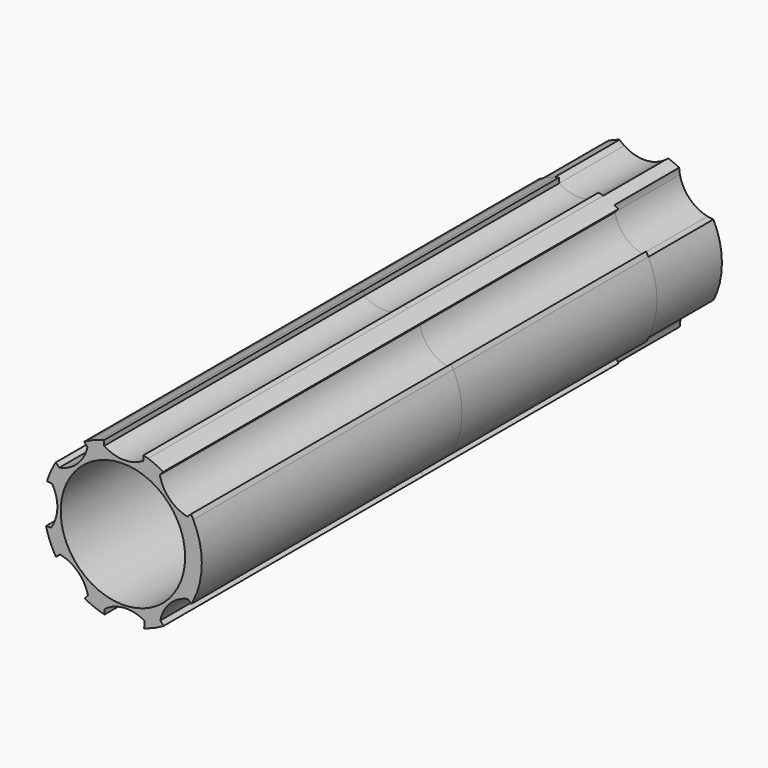
from build123d import *

# Parameters (mm, degrees)
F0_R          = 4.8612376023
F1_DEPTH      = 25.4
F1_DEPTH_BACK = 25.4
F2_DEPTH      = 19.05
F2_DEPTH_BACK = 25.4
F3_DEPTH      = 25.4
F3_DEPTH_BACK = 25.4
F4_T2_ANGLE   = 271.2368100282


# Not quite as in the source:
# - a fillet or chamfer that OpenCascade refuses, or shapes differently, is made with other operations: its cross-section is extruded or revolved along the edge and cut away or added


with BuildPart() as f1:
    # F0 (on Front) → F1 (new body, two sides)
    with BuildSketch(Plane.XZ) as f1_sk:
        with BuildLine():
            ThreePointArc((-5.6143828163, -1.3793864731), (-5.7555397167, -1.5672020545), (-5.9119525631, -1.7425160147))
            ThreePointArc((-5.9119525631, -1.7425160147), (-5.6940196105, -2.3591705842), (-5.4119693183, -2.9492597831))
            ThreePointArc((-5.4119693183, -2.9492597831), (-5.1782834381, -2.962493255), (-4.9465206336, -2.9952074382))
            ThreePointArc((-4.9465206336, -2.9952074382), (-3.5276076708, -3.7167374387), (-2.7316714584, -5.0952892453))
            ThreePointArc((-2.7316714584, -5.0952892453), (-2.6865496833, -5.3258624193), (-2.6609266437, -5.5594077533))
            ThreePointArc((-2.6609266437, -5.5594077533), (-2.2164022319, -5.751096097), (-1.7582047643, -5.907305746))
            ThreePointArc((-1.7582047643, -5.907305746), (-1.5960910736, -5.7494322847), (-1.4217527636, -5.6051719916))
            ThreePointArc((-1.4217527636, -5.6051719916), (0.114197137, -5.0376327164), (1.7047800347, -5.4265915467))
            Line((1.7047800347, -5.4265915467), (1.6597306544, -5.935725678))
            ThreePointArc((1.6597306544, -5.935725678), (2.2765492286, -5.7275534725), (2.8679699144, -5.4554829062))
            ThreePointArc((2.8679699144, -5.4554829062), (2.8846977078, -5.22202114), (2.9208752645, -4.990773654))
            ThreePointArc((2.9208752645, -4.990773654), (3.6635506236, -3.582813126), (5.0538549065, -2.807588295))
            ThreePointArc((5.0538549065, -2.807588295), (5.2850772748, -2.7659208069), (5.5189797809, -2.7437943341))
            ThreePointArc((5.5189797809, -2.7437943341), (6.1633583889, 0.023633466), (5.4977755768, 2.7860382045))
            ThreePointArc((5.4977755768, 2.7860382045), (5.2645901724, 2.8062565756), (5.0339097574, 2.8458894094))
            ThreePointArc((5.0339097574, 2.8458894094), (3.6372167606, 3.6095439191), (2.8828768034, 5.0112895332))
            ThreePointArc((2.8828768034, 5.0112895332), (2.8446729274, 5.2431093491), (2.8260479734, 5.4773166809))
            ThreePointArc((2.8260479734, 5.4773166809), (2.4006224975, 5.6766677545), (1.961248138, 5.8430343924))
            ThreePointArc((1.961248138, 5.8430343924), (1.7809432193, 5.6937884489), (1.588797766, 5.5601309009))
            ThreePointArc((1.588797766, 5.5601309009), (0.0578959269, 5.1239439038), (-1.4632199599, 5.5931197733))
            ThreePointArc((-1.4632199599, 5.5931197733), (-1.6531261487, 5.7314512688), (-1.830760335, 5.88522402))
            ThreePointArc((-1.830760335, 5.88522402), (-2.2737274404, 5.728674253), (-2.7034829894, 5.5388378651))
            ThreePointArc((-2.7034829894, 5.5388378651), (-2.7271874135, 5.3059810086), (-2.7702666546, 5.07591929))
            ThreePointArc((-2.7702666546, 5.07591929), (-3.5547294118, 3.6908063992), (-4.9676026515, 2.9575201346))
            ThreePointArc((-4.9676026515, 2.9575201346), (-5.1999680345, 2.9227884204), (-5.4344277772, 2.9076691533))
            ThreePointArc((-5.4344277772, 2.9076691533), (-5.6401206566, 2.4852734556), (-5.8130414583, 2.0484370076))
            ThreePointArc((-5.8130414583, 2.0484370076), (-5.6665094698, 1.8659196339), (-5.5357412598, 1.6717962436))
            ThreePointArc((-5.5357412598, 1.6717962436), (-5.122504455, 0.1345406108), (-5.6143828163, -1.3793864731))
        make_face()
        Circle(F0_R, mode=Mode.SUBTRACT)
    extrude(amount=-F1_DEPTH)
    extrude(f1_sk.sketch, amount=F1_DEPTH_BACK)

    # F0 (on Front) → F2 (join, two sides)
    with BuildSketch(Plane.XZ) as f2_sk:
        with BuildLine():
            ThreePointArc((3.1433341705, 5.3016031031), (2.9859838597, 5.3917942802), (2.8260479734, 5.4773166809))
            ThreePointArc((2.8260479734, 5.4773166809), (2.8446729274, 5.2431093491), (2.8828768034, 5.0112895332))
            Line((2.8828768034, 5.0112895332), (3.1433341705, 5.3016031031))
        make_face()
        with BuildLine():
            Line((1.6092045641, 5.9496223276), (1.588797766, 5.5601309009))
            ThreePointArc((1.588797766, 5.5601309009), (1.7809432193, 5.6937884489), (1.961248138, 5.8430343924))
            ThreePointArc((1.961248138, 5.8430343924), (1.7860216604, 5.8989551447), (1.6092045641, 5.9496223276))
        make_face()
        with BuildLine():
            ThreePointArc((-1.4814178118, 5.9827206551), (-1.6568063911, 5.9365425757), (-1.830760335, 5.88522402))
            ThreePointArc((-1.830760335, 5.88522402), (-1.6531261487, 5.7314512688), (-1.4632199599, 5.5931197733))
            Line((-1.4632199599, 5.5931197733), (-1.4814178118, 5.9827206551))
        make_face()
        with BuildLine():
            Line((-3.0290736059, 5.3677051205), (-2.7702666546, 5.07591929))
            ThreePointArc((-2.7702666546, 5.07591929), (-2.7271874135, 5.3059810086), (-2.7034829894, 5.5388378651))
            ThreePointArc((-2.7034829894, 5.5388378651), (-2.8675552102, 5.4557008978), (-3.0290736059, 5.3677051205))
        make_face()
        with BuildLine():
            ThreePointArc((-5.253987448, 3.2222912758), (-5.3465224003, 3.0663077787), (-5.4344277772, 2.9076691533))
            ThreePointArc((-5.4344277772, 2.9076691533), (-5.1999680345, 2.9227884204), (-4.9676026515, 2.9575201346))
            Line((-4.9676026515, 2.9575201346), (-5.253987448, 3.2222912758))
        make_face()
        with BuildLine():
            Line((-5.9248838296, 1.698027319), (-5.5357412598, 1.6717962436))
            ThreePointArc((-5.5357412598, 1.6717962436), (-5.6665094698, 1.8659196339), (-5.8130414583, 2.0484370076))
            ThreePointArc((-5.8130414583, 2.0484370076), (-5.8715772373, 1.8740666788), (-5.9248838296, 1.698027319))
        make_face()
        with BuildLine():
            ThreePointArc((-6.0042123315, -1.3917540905), (-5.9606631284, -1.5678138408), (-5.9119525631, -1.7425160147))
            ThreePointArc((-5.9119525631, -1.7425160147), (-5.7555397167, -1.5672020545), (-5.6143828163, -1.3793864731))
            Line((-5.6143828163, -1.3793864731), (-6.0042123315, -1.3917540905))
        make_face()
        with BuildLine():
            ThreePointArc((5.0339097574, 2.8458894094), (5.2645901724, 2.8062565756), (5.4977755768, 2.7860382045))
            ThreePointArc((5.4977755768, 2.7860382045), (5.4121934892, 2.9488483863), (5.321791339, 3.1090323437))
            Line((5.321791339, 3.1090323437), (5.0339097574, 2.8458894094))
        make_face()
        with BuildLine():
            ThreePointArc((5.5189797809, -2.7437943341), (5.2850772748, -2.7659208069), (5.0538549065, -2.807588295))
            Line((5.0538549065, -2.807588295), (5.3480322785, -3.0636735985))
            ThreePointArc((5.3480322785, -3.0636735985), (5.4358594961, -2.9049916883), (5.5189797809, -2.7437943341))
        make_face()
        with BuildLine():
            ThreePointArc((2.9208752645, -4.990773654), (2.8846977078, -5.22202114), (2.8679699144, -5.4554829062))
            ThreePointArc((2.8679699144, -5.4554829062), (3.0294816207, -5.3674748514), (3.1882952913, -5.27468656))
            Line((3.1882952913, -5.27468656), (2.9208752645, -4.990773654))
        make_face()
        with BuildLine():
            ThreePointArc((-5.6143828163, -1.3793864731), (-5.7555397167, -1.5672020545), (-5.9119525631, -1.7425160147))
            ThreePointArc((-5.9119525631, -1.7425160147), (-5.6940196105, -2.3591705842), (-5.4119693183, -2.9492597831))
            ThreePointArc((-5.4119693183, -2.9492597831), (-5.1782834381, -2.962493255), (-4.9465206336, -2.9952074382))
            ThreePointArc((-4.9465206336, -2.9952074382), (-3.5276076708, -3.7167374387), (-2.7316714584, -5.0952892453))
            ThreePointArc((-2.7316714584, -5.0952892453), (-2.6865496833, -5.3258624193), (-2.6609266437, -5.5594077533))
            ThreePointArc((-2.6609266437, -5.5594077533), (-2.2164022319, -5.751096097), (-1.7582047643, -5.907305746))
            ThreePointArc((-1.7582047643, -5.907305746), (-1.5960910736, -5.7494322847), (-1.4217527636, -5.6051719916))
            ThreePointArc((-1.4217527636, -5.6051719916), (0.114197137, -5.0376327164), (1.7047800347, -5.4265915467))
            Line((1.7047800347, -5.4265915467), (1.6597306544, -5.935725678))
            ThreePointArc((1.6597306544, -5.935725678), (2.2765492286, -5.7275534725), (2.8679699144, -5.4554829062))
            ThreePointArc((2.8679699144, -5.4554829062), (2.8846977078, -5.22202114), (2.9208752645, -4.990773654))
            ThreePointArc((2.9208752645, -4.990773654), (3.6635506236, -3.582813126), (5.0538549065, -2.807588295))
            ThreePointArc((5.0538549065, -2.807588295), (5.2850772748, -2.7659208069), (5.5189797809, -2.7437943341))
            ThreePointArc((5.5189797809, -2.7437943341), (6.1633583889, 0.023633466), (5.4977755768, 2.7860382045))
            ThreePointArc((5.4977755768, 2.7860382045), (5.2645901724, 2.8062565756), (5.0339097574, 2.8458894094))
            ThreePointArc((5.0339097574, 2.8458894094), (3.6372167606, 3.6095439191), (2.8828768034, 5.0112895332))
            ThreePointArc((2.8828768034, 5.0112895332), (2.8446729274, 5.2431093491), (2.8260479734, 5.4773166809))
            ThreePointArc((2.8260479734, 5.4773166809), (2.4006224975, 5.6766677545), (1.961248138, 5.8430343924))
            ThreePointArc((1.961248138, 5.8430343924), (1.7809432193, 5.6937884489), (1.588797766, 5.5601309009))
            ThreePointArc((1.588797766, 5.5601309009), (0.0578959269, 5.1239439038), (-1.4632199599, 5.5931197733))
            ThreePointArc((-1.4632199599, 5.5931197733), (-1.6531261487, 5.7314512688), (-1.830760335, 5.88522402))
            ThreePointArc((-1.830760335, 5.88522402), (-2.2737274404, 5.728674253), (-2.7034829894, 5.5388378651))
            ThreePointArc((-2.7034829894, 5.5388378651), (-2.7271874135, 5.3059810086), (-2.7702666546, 5.07591929))
            ThreePointArc((-2.7702666546, 5.07591929), (-3.5547294118, 3.6908063992), (-4.9676026515, 2.9575201346))
            ThreePointArc((-4.9676026515, 2.9575201346), (-5.1999680345, 2.9227884204), (-5.4344277772, 2.9076691533))
            ThreePointArc((-5.4344277772, 2.9076691533), (-5.6401206566, 2.4852734556), (-5.8130414583, 2.0484370076))
            ThreePointArc((-5.8130414583, 2.0484370076), (-5.6665094698, 1.8659196339), (-5.5357412598, 1.6717962436))
            ThreePointArc((-5.5357412598, 1.6717962436), (-5.122504455, 0.1345406108), (-5.6143828163, -1.3793864731))
        make_face()
        Circle(F0_R, mode=Mode.SUBTRACT)
        with BuildLine():
            ThreePointArc((-1.4217527636, -5.6051719916), (-1.5960910736, -5.7494322847), (-1.7582047643, -5.907305746))
            ThreePointArc((-1.7582047643, -5.907305746), (-1.5949558747, -5.9534578967), (-1.4304986106, -5.9950995734))
            Line((-1.4304986106, -5.9950995734), (-1.4217527636, -5.6051719916))
        make_face()
        with BuildLine():
            ThreePointArc((-2.6609266437, -5.5594077533), (-2.6865496833, -5.3258624193), (-2.7316714584, -5.0952892453))
            Line((-2.7316714584, -5.0952892453), (-2.9833273874, -5.3932645837))
            ThreePointArc((-2.9833273874, -5.3932645837), (-2.8233493903, -5.4787081863), (-2.6609266437, -5.5594077533))
        make_face()
        with BuildLine():
            ThreePointArc((-4.9465206336, -2.9952074382), (-5.1782834381, -2.962493255), (-5.4119693183, -2.9492597831))
            ThreePointArc((-5.4119693183, -2.9492597831), (-5.321554992, -3.1094368681), (-5.2264013251, -3.2668447099))
            Line((-5.2264013251, -3.2668447099), (-4.9465206336, -2.9952074382))
        make_face()
    extrude(amount=-F2_DEPTH)
    extrude(f2_sk.sketch, amount=F2_DEPTH_BACK)


with BuildPart() as f3:
    # F0 (on Front) → F3 (new body, two sides)
    with BuildSketch(Plane.XZ) as f3_sk:
        with BuildLine():
            Line((-1.3347425842, -5.6051719916), (-1.3347425842, -5.8972059093))
            ThreePointArc((-1.3347425842, -5.8972059093), (0.1551903565, -6.0448676148), (1.63668259, -5.8283383814))
            Line((1.63668259, -5.8283383814), (1.6722300908, -5.4265915467))
            ThreePointArc((1.6722300908, -5.4265915467), (0.1408736066, -5.0465987547), (-1.3347425842, -5.6051719916))
        make_face()
    extrude(amount=-F3_DEPTH)
    extrude(f3_sk.sketch, amount=F3_DEPTH_BACK)

    # F4: chamfer of 5.08 on 1 edges, made by hand

    # F4_s1 → F4_t2 (revolve, cut)
    with BuildSketch(Plane(origin=(0.0596949871, 0, 0.0611915478), x_dir=(0, 1, 0), z_dir=(0.6982993759, 0, 0.7158058268))):
        Polygon((-20.32, 6.219428276), (-25.4, 1.139428276), (-25.4, 6.219428276), align=None)
    revolve(axis=Axis((0.0126080508, -25.4, 0.1071268796), (0, -1, 0)), revolution_arc=F4_T2_ANGLE, mode=Mode.SUBTRACT)


solid = Compound([f1.part, f3.part])
